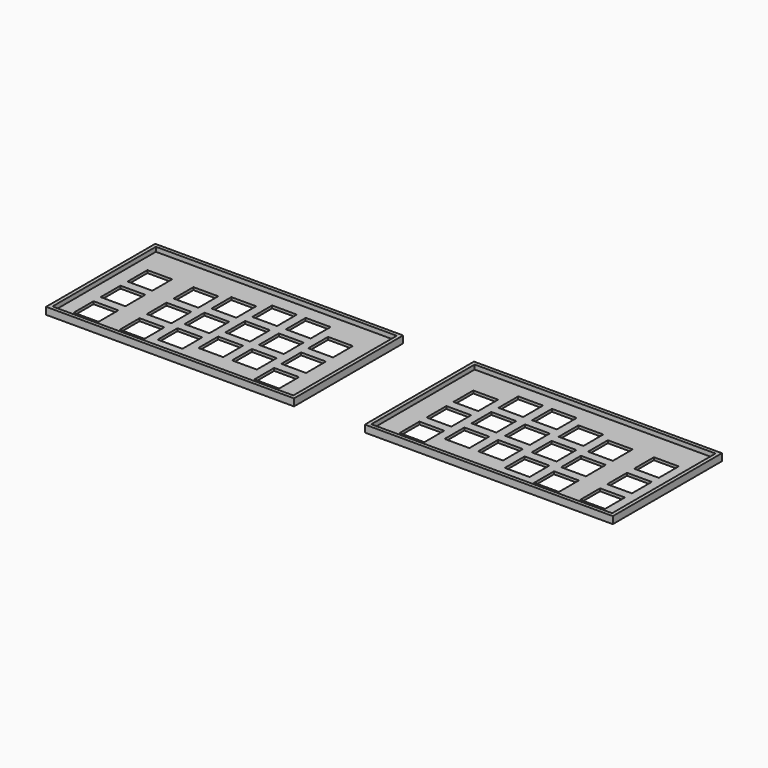
from build123d import *

# Parameters (mm, degrees)
F1_DEPTH = 1.5
F3_DEPTH = 25
F4_DEPTH = 4


# Not quite as in the source:
# - a feature names something its author has since deleted; it is built from what else it names


with BuildPart() as f1:
    # F0 (on Top) → F1 (new body)
    with BuildSketch(Plane.XY):
        Polygon((-9.6456400305, -38.5), (70, -38.5), (70, -5.2260886878), (68, -5.2260886878), (68, -36.5), (-9.6456400305, -36.5), align=None)
        Polygon((-70, -38.5), (-9.6456400305, -38.5), (-9.6456400305, -36.5), (-68, -36.5), (-68, 2.6378679238), (-70, 2.6378679238), align=None)
        Polygon((-70, 38.5), (-70, 2.6378679238), (-68, 2.6378679238), (-68, 36.5), (-20.2697571367, 36.5), (-20.2697571367, 38.5), align=None)
        Polygon((68, -5.2260886878), (70, -5.2260886878), (70, 38.5), (-20.2697571367, 38.5), (-20.2697571367, 36.5), (68, 36.5), align=None)
        Polygon((-68, -36.5), (-9.6456400305, -36.5), (68, -36.5), (68, -5.2260886878), (68, 36.5), (-20.2697571367, 36.5), (-68, 36.5), (-68, 2.6378679238), align=None)
    extrude(amount=F1_DEPTH)

    # F2 (on face) → F3 (cut)
    with BuildSketch(Plane.XY.offset(1.5)):
        Polygon((56, -17.5), (49, -17.5), (42, -17.5), (42, -31.5), (56, -31.5), align=None)
        Polygon((-1, 23.5), (-8, 23.5), (-15, 23.5), (-15, 17.9919603638), (-15, 9.5), (-8, 9.5), (-1, 9.5), (-1, 14.5402538426), align=None)
        Polygon((-1, 4.5), (-8, 4.5), (-15, 4.5), (-15, -1.0080396362), (-15, -9.5), (-8, -9.5), (-1, -9.5), (-1, 0.6484970983), align=None)
        Polygon((-1, -14.5), (-8, -14.5), (-15, -14.5), (-15, -14.8997963805), (-15, -28.5), (-1, -28.5), align=None)
        Polygon((18, 28.5), (11, 28.5), (4, 28.5), (4, 14.5402538426), (4, 14.5), (11, 14.5), (18, 14.5), (18, 19.3217483706), align=None)
        Polygon((18, 9.5), (11, 9.5), (4, 9.5), (4, -4.5), (11, -4.5), (18, -4.5), (18, 0.3217483706), align=None)
        Polygon((18, -9.5), (11, -9.5), (4, -9.5), (4, -23.5), (18, -23.5), (18, -13.5700083736), align=None)
        Polygon((37, -9.5), (30, -9.5), (23, -9.5), (23, -23.5), (37, -23.5), align=None)
        Polygon((56, 1.5), (49, 1.5), (42, 1.5), (42, -12.5), (49, -12.5), (56, -12.5), align=None)
        Polygon((56, 20.5), (49, 20.5), (42, 20.5), (42, 20.1662803835), (42, 6.5), (49, 6.5), (56, 6.5), align=None)
        Polygon((-53, 6.5), (-46, 6.5), (-46, 20.5), (-53, 20.5), (-60, 20.5), (-60, 6.5), align=None)
        Polygon((-46, -17.5), (-53, -17.5), (-60, -17.5), (-60, -31.5), (-46, -31.5), align=None)
        Polygon((-46, 1.5), (-53, 1.5), (-60, 1.5), (-60, -12.5), (-53, -12.5), (-46, -12.5), align=None)
        Polygon((-20, -17.5), (-27, -17.5), (-34, -17.5), (-34, -31.5), (-20, -31.5), align=None)
        Polygon((-20, 20.5), (-27, 20.5), (-34, 20.5), (-34, 6.5), (-27, 6.5), (-20, 6.5), (-20, 17.9919603638), align=None)
        Polygon((-20, 1.5), (-27, 1.5), (-34, 1.5), (-34, -12.5), (-27, -12.5), (-20, -12.5), (-20, -1.0080396362), align=None)
        Polygon((37, 28.5), (30, 28.5), (23, 28.5), (23, 19.3217483706), (23, 14.5), (30, 14.5), (37, 14.5), (37, 20.1662803835), align=None)
        Polygon((37, 9.5), (30, 9.5), (23, 9.5), (23, 0.3217483706), (23, -4.5), (30, -4.5), (37, -4.5), (37, 6.2745236393), align=None)
    extrude(amount=-F3_DEPTH, mode=Mode.SUBTRACT)

    # F0 (on Top) → F4 (join)
    with BuildSketch(Plane.XY):
        Polygon((-9.6456400305, -38.5), (70, -38.5), (70, -5.2260886878), (68, -5.2260886878), (68, -36.5), (-9.6456400305, -36.5), align=None)
        Polygon((-70, -38.5), (-9.6456400305, -38.5), (-9.6456400305, -36.5), (-68, -36.5), (-68, 2.6378679238), (-70, 2.6378679238), align=None)
        Polygon((68, -5.2260886878), (70, -5.2260886878), (70, 38.5), (-20.2697571367, 38.5), (-20.2697571367, 36.5), (68, 36.5), align=None)
        Polygon((-70, 38.5), (-70, 2.6378679238), (-68, 2.6378679238), (-68, 36.5), (-20.2697571367, 36.5), (-20.2697571367, 38.5), align=None)
    extrude(amount=F4_DEPTH)


with BuildPart() as f6_1:
    # F6: instance of F1
    add(f1.part.mirror(Plane.YZ.offset(90)))


solid = Compound([f1.part, f6_1.part])
